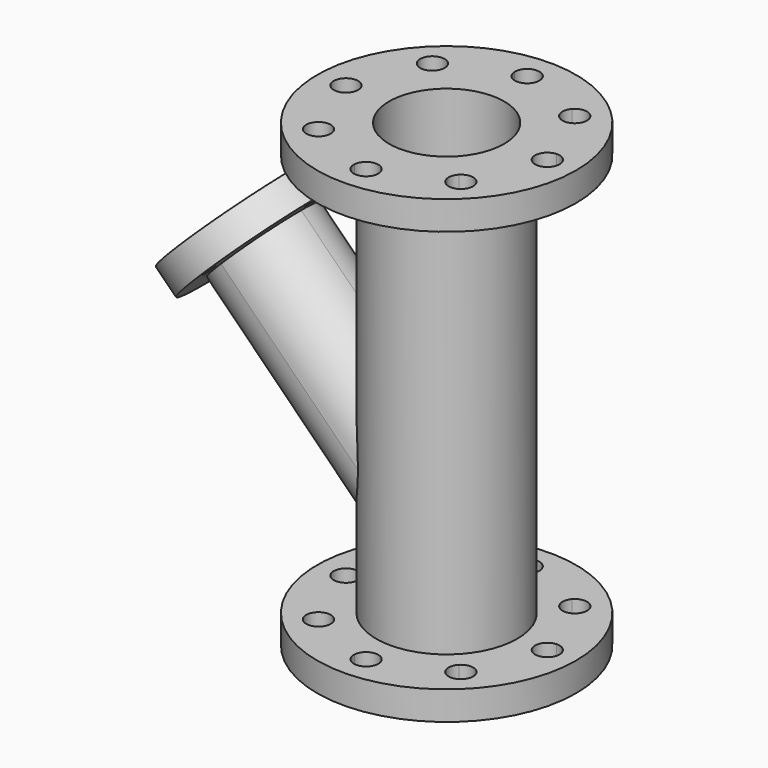
from build123d import *

# Parameters (mm, degrees)
F0_R      = 45
F1_DEPTH  = 10
F2_R      = 24.5
F2_R_2    = 20
F3_DEPTH  = 140
F4_R      = 45
F4_R_2    = 24.5
F4_R_3    = 20
F5_DEPTH  = 10
F8_DEPTH  = 195
F10_DEPTH = 18.5
F11_R     = 18.499
F12_R     = 28.5
F13_DEPTH = 10
F15_DEPTH = 25
F16_R     = 14
F17_DEPTH = 99.7
F18_R     = 20
F19_DEPTH = 202.6


# Not quite as in the source:
# - a fillet or chamfer is up to 0.001 mm smaller than in the source, because OpenCascade refuses the exact size


with BuildPart() as f1:
    # F0 (on Top) → F1 (new body)
    with BuildSketch(Plane.XY):
        Circle(F0_R)
    extrude(amount=F1_DEPTH)

    # F2 (on face) → F3 (join)
    with BuildSketch(Plane.XY.offset(10)):
        Circle(F2_R)
        Circle(F2_R_2, mode=Mode.SUBTRACT)
        Circle(F2_R_2)
    extrude(amount=F3_DEPTH)

    # F4 (on face) → F5 (join)
    with BuildSketch(Plane.XY.offset(150)):
        Circle(F4_R)
        Circle(F4_R_2, mode=Mode.SUBTRACT)
        Circle(F4_R_2)
        Circle(F4_R_3, mode=Mode.SUBTRACT)
        Circle(F4_R_3)
    extrude(amount=F5_DEPTH)

    # F7 (on face) → F8 (cut)
    with BuildSketch(Plane(origin=(0, 0, 0), x_dir=(1, 0, 0), z_dir=(0, 0, -1))):
        with BuildLine():
            ThreePointArc((-34.7419642857, -4.2421595409), (-35, 0), (-34.7419642857, 4.2421595409))
            ThreePointArc((-34.7419642857, 4.2421595409), (-39.25, 0), (-34.7419642857, -4.2421595409))
        make_face()
        with BuildLine():
            ThreePointArc((-30.75, 0), (-31.904911004, 2.9125459837), (-34.7419642857, 4.2421595409))
            ThreePointArc((-34.7419642857, 4.2421595409), (-35, 0), (-34.7419642857, -4.2421595409))
            ThreePointArc((-34.7419642857, -4.2421595409), (-31.904911004, -2.9125459837), (-30.75, 0))
        make_face()
        with BuildLine():
            ThreePointArc((-4.2421595409, -34.7419642857), (0, -35), (4.2421595409, -34.7419642857))
            ThreePointArc((4.2421595409, -34.7419642857), (0, -30.75), (-4.2421595409, -34.7419642857))
        make_face()
        with BuildLine():
            ThreePointArc((4.25, -35), (4.248039433, -34.8709225982), (4.2421595409, -34.7419642857))
            ThreePointArc((4.2421595409, -34.7419642857), (0, -35), (-4.2421595409, -34.7419642857))
            ThreePointArc((-4.2421595409, -34.7419642857), (-0.1290774018, -39.248039433), (4.25, -35))
        make_face()
        with BuildLine():
            ThreePointArc((34.7419642857, -4.2421595409), (34.935431513, -2.125), (35, 0))
            ThreePointArc((35, 0), (34.935431513, 2.125), (34.7419642857, 4.2421595409))
            ThreePointArc((34.7419642857, 4.2421595409), (30.75, 0), (34.7419642857, -4.2421595409))
        make_face()
        with BuildLine():
            ThreePointArc((34.7419642857, 4.2421595409), (34.935431513, 2.125), (35, 0))
            ThreePointArc((35, 0), (34.935431513, -2.125), (34.7419642857, -4.2421595409))
            ThreePointArc((34.7419642857, -4.2421595409), (37.9125459837, -3.095088996), (39.25, 0))
            ThreePointArc((39.25, 0), (37.9125459837, 3.095088996), (34.7419642857, 4.2421595409))
        make_face()
        with BuildLine():
            ThreePointArc((24.7487373415, 24.7487373415), (26.2056824365, 23.2004786165), (27.5659383164, 21.5666187599))
            ThreePointArc((27.5659383164, 21.5666187599), (28.6240182438, 23.0038310608), (28.9987373415, 24.7487373415))
            ThreePointArc((28.9987373415, 24.7487373415), (26.2551396829, 28.7228098102), (21.5666187599, 27.5659383164))
            ThreePointArc((21.5666187599, 27.5659383164), (23.2004786165, 26.2056824365), (24.7487373415, 24.7487373415))
        make_face()
        with BuildLine():
            ThreePointArc((21.7435335215, 21.7435335215), (24.6196599397, 20.5006979085), (27.5659383164, 21.5666187599))
            ThreePointArc((27.5659383164, 21.5666187599), (26.2056824365, 23.2004786165), (24.7487373415, 24.7487373415))
            Line((24.7487373415, 24.7487373415), (21.7435335215, 21.7435335215))
        make_face()
        with BuildLine():
            Line((21.7435335215, 21.7435335215), (24.7487373415, 24.7487373415))
            ThreePointArc((24.7487373415, 24.7487373415), (23.2004786165, 26.2056824365), (21.5666187599, 27.5659383164))
            ThreePointArc((21.5666187599, 27.5659383164), (20.5006979085, 24.6196599397), (21.7435335215, 21.7435335215))
        make_face()
        with BuildLine():
            ThreePointArc((28.9987373415, -24.7487373415), (28.6240182438, -23.0038310608), (27.5659383164, -21.5666187599))
            ThreePointArc((27.5659383164, -21.5666187599), (26.2056824365, -23.2004786165), (24.7487373415, -24.7487373415))
            ThreePointArc((24.7487373415, -24.7487373415), (23.2004786165, -26.2056824365), (21.5666187599, -27.5659383164))
            ThreePointArc((21.5666187599, -27.5659383164), (26.2551396829, -28.7228098102), (28.9987373415, -24.7487373415))
        make_face()
        with BuildLine():
            ThreePointArc((21.5666187599, -27.5659383164), (23.2004786165, -26.2056824365), (24.7487373415, -24.7487373415))
            Line((24.7487373415, -24.7487373415), (21.7435335215, -21.7435335215))
            ThreePointArc((21.7435335215, -21.7435335215), (20.5006979085, -24.6196599397), (21.5666187599, -27.5659383164))
        make_face()
        with BuildLine():
            ThreePointArc((24.7487373415, -24.7487373415), (26.2056824365, -23.2004786165), (27.5659383164, -21.5666187599))
            ThreePointArc((27.5659383164, -21.5666187599), (24.6196599397, -20.5006979085), (21.7435335215, -21.7435335215))
            Line((21.7435335215, -21.7435335215), (24.7487373415, -24.7487373415))
        make_face()
        with BuildLine():
            ThreePointArc((-27.5659383164, -21.5666187599), (-27.7539411616, -27.7539411616), (-21.5666187599, -27.5659383164))
            ThreePointArc((-21.5666187599, -27.5659383164), (-23.2004786165, -26.2056824365), (-24.7487373415, -24.7487373415))
            ThreePointArc((-24.7487373415, -24.7487373415), (-26.2056824365, -23.2004786165), (-27.5659383164, -21.5666187599))
        make_face()
        with BuildLine():
            Line((-24.7487373415, -24.7487373415), (-21.7435335215, -21.7435335215))
            ThreePointArc((-21.7435335215, -21.7435335215), (-24.6196599397, -20.5006979085), (-27.5659383164, -21.5666187599))
            ThreePointArc((-27.5659383164, -21.5666187599), (-26.2056824365, -23.2004786165), (-24.7487373415, -24.7487373415))
        make_face()
        with BuildLine():
            ThreePointArc((-20.4987373415, -24.7487373415), (-20.8222493284, -23.122332754), (-21.7435335215, -21.7435335215))
            Line((-21.7435335215, -21.7435335215), (-24.7487373415, -24.7487373415))
            ThreePointArc((-24.7487373415, -24.7487373415), (-23.2004786165, -26.2056824365), (-21.5666187599, -27.5659383164))
            ThreePointArc((-21.5666187599, -27.5659383164), (-20.7746648729, -26.2551396829), (-20.4987373415, -24.7487373415))
        make_face()
        with BuildLine():
            ThreePointArc((-24.7487373415, 24.7487373415), (-23.2004786165, 26.2056824365), (-21.5666187599, 27.5659383164))
            ThreePointArc((-21.5666187599, 27.5659383164), (-27.7539411616, 27.7539411616), (-27.5659383164, 21.5666187599))
            ThreePointArc((-27.5659383164, 21.5666187599), (-26.2056824365, 23.2004786165), (-24.7487373415, 24.7487373415))
        make_face()
        with BuildLine():
            ThreePointArc((-20.4987373415, 24.7487373415), (-20.7746648729, 26.2551396829), (-21.5666187599, 27.5659383164))
            ThreePointArc((-21.5666187599, 27.5659383164), (-23.2004786165, 26.2056824365), (-24.7487373415, 24.7487373415))
            Line((-24.7487373415, 24.7487373415), (-21.7435335215, 21.7435335215))
            ThreePointArc((-21.7435335215, 21.7435335215), (-20.8222493284, 23.122332754), (-20.4987373415, 24.7487373415))
        make_face()
        with BuildLine():
            ThreePointArc((-27.5659383164, 21.5666187599), (-24.6196599397, 20.5006979085), (-21.7435335215, 21.7435335215))
            Line((-21.7435335215, 21.7435335215), (-24.7487373415, 24.7487373415))
            ThreePointArc((-24.7487373415, 24.7487373415), (-26.2056824365, 23.2004786165), (-27.5659383164, 21.5666187599))
        make_face()
        with BuildLine():
            ThreePointArc((-4.2421595409, 34.7419642857), (0, 30.75), (4.2421595409, 34.7419642857))
            ThreePointArc((4.2421595409, 34.7419642857), (0, 35), (-4.2421595409, 34.7419642857))
        make_face()
        with BuildLine():
            ThreePointArc((-4.2421595409, 34.7419642857), (0, 35), (4.2421595409, 34.7419642857))
            ThreePointArc((4.2421595409, 34.7419642857), (4.248039433, 34.8709225982), (4.25, 35))
            ThreePointArc((4.25, 35), (-0.1290774018, 39.248039433), (-4.2421595409, 34.7419642857))
        make_face()
    extrude(amount=-F8_DEPTH, mode=Mode.SUBTRACT)

    # F9 (on Front) → F10 (join, symmetric)
    with BuildSketch(Plane.XZ):
        Polygon((-76.7210857587, 90.5581348548), (0, 13.8370490961), (0, 40), (-63.6396103068, 103.6396103068), align=None)
        Polygon((0, 40), (0, 13.8370490961), (6.2413537338, 59.9215971701), (0, 66.1629509039), align=None)
        Polygon((-63.6396103068, 103.6396103068), (0, 40), (0, 66.1629509039), (-50.5581348548, 116.7210857587), align=None)
    extrude(amount=F10_DEPTH, both=True)

    # F11 (radius 18.5 in the source; OpenCascade refuses exactly that, so slightly less here)
    f11_edges = [f1.edges().sort_by_distance(p)[0] for p in [
        (-46.391732, 18.5, 60.228781),
        (-46.391732, -18.5, 60.228781),
        (-33.310257, -18.5, 99.473208),
        (-33.310257, 18.5, 99.473208),
    ]]
    fillet(f11_edges, radius=F11_R)

    # F12 (on face) → F13 (join)
    with BuildSketch(Plane(origin=(-83.6396103068, 0, 83.6396103068), x_dir=(0, -1, 0), z_dir=(-0.7071067812, 0, 0.7071067812))):
        with Locations((0, 28.2842712475)):
            Circle(F12_R)
    extrude(amount=F13_DEPTH)

    # F14 (on face) → F15 (cut)
    with BuildSketch(Plane(origin=(-90.7106781187, 0, 90.7106781187), x_dir=(0, -1, 0), z_dir=(-0.7071067812, 0, 0.7071067812))):
        with BuildLine():
            ThreePointArc((-2.24742029, 51.6765584815), (0, 49.5342712475), (2.24742029, 51.6765584815))
            ThreePointArc((2.24742029, 51.6765584815), (0, 51.7842712475), (-2.24742029, 51.6765584815))
        make_face()
        with BuildLine():
            ThreePointArc((-2.24742029, 51.6765584815), (0, 51.7842712475), (2.24742029, 51.6765584815))
            ThreePointArc((2.24742029, 51.6765584815), (2.2493549801, 51.7303994207), (2.25, 51.7842712475))
            ThreePointArc((2.25, 51.7842712475), (-0.0538718267, 54.0336262275), (-2.24742029, 51.6765584815))
        make_face()
        with BuildLine():
            ThreePointArc((-23.392287234, 26.0368509574), (-23.5, 28.2842712475), (-23.392287234, 30.5316915375))
            ThreePointArc((-23.392287234, 30.5316915375), (-25.75, 28.2842712475), (-23.392287234, 26.0368509574))
        make_face()
        with BuildLine():
            ThreePointArc((-21.25, 28.2842712475), (-21.8713727063, 29.8367122732), (-23.392287234, 30.5316915375))
            ThreePointArc((-23.392287234, 30.5316915375), (-23.5, 28.2842712475), (-23.392287234, 26.0368509574))
            ThreePointArc((-23.392287234, 26.0368509574), (-21.8713727063, 26.7318302218), (-21.25, 28.2842712475))
        make_face()
        with BuildLine():
            ThreePointArc((-2.24742029, 4.8919840134), (0, 4.7842712475), (2.24742029, 4.8919840134))
            ThreePointArc((2.24742029, 4.8919840134), (0, 7.0342712475), (-2.24742029, 4.8919840134))
        make_face()
        with BuildLine():
            ThreePointArc((2.25, 4.7842712475), (2.2493549801, 4.8381430742), (2.24742029, 4.8919840134))
            ThreePointArc((2.24742029, 4.8919840134), (0, 4.7842712475), (-2.24742029, 4.8919840134))
            ThreePointArc((-2.24742029, 4.8919840134), (-0.0538718267, 2.5349162674), (2.25, 4.7842712475))
        make_face()
        with BuildLine():
            ThreePointArc((23.392287234, 26.0368509574), (23.4730563626, 27.1592712475), (23.5, 28.2842712475))
            ThreePointArc((23.5, 28.2842712475), (23.4730563626, 29.4092712475), (23.392287234, 30.5316915375))
            ThreePointArc((23.392287234, 30.5316915375), (21.25, 28.2842712475), (23.392287234, 26.0368509574))
        make_face()
        with BuildLine():
            ThreePointArc((23.392287234, 30.5316915375), (23.4730563626, 29.4092712475), (23.5, 28.2842712475))
            ThreePointArc((23.5, 28.2842712475), (23.4730563626, 27.1592712475), (23.392287234, 26.0368509574))
            ThreePointArc((23.392287234, 26.0368509574), (25.0524410257, 26.6556439538), (25.75, 28.2842712475))
            ThreePointArc((25.75, 28.2842712475), (25.0524410257, 29.9128985411), (23.392287234, 30.5316915375))
        make_face()
    extrude(amount=-F15_DEPTH, mode=Mode.SUBTRACT)

    # F16 (on face) → F17 (cut)
    with BuildSketch(Plane(origin=(-90.7106781187, 0, 90.7106781187), x_dir=(0, -1, 0), z_dir=(-0.7071067812, 0, 0.7071067812))):
        with Locations((0, 28.2842712475)):
            Circle(F16_R)
    extrude(amount=-F17_DEPTH, mode=Mode.SUBTRACT)

    # F18 (on face) → F19 (cut)
    with BuildSketch(Plane.XY.offset(160)):
        Circle(F18_R)
    extrude(amount=-F19_DEPTH, mode=Mode.SUBTRACT)


solid = f1.part
